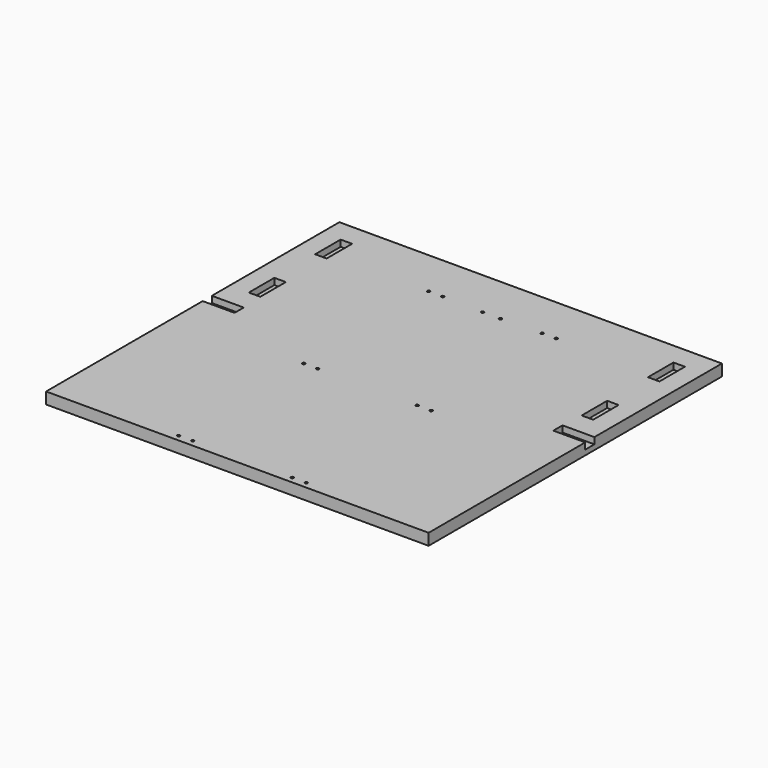
from build123d import *

# Parameters (mm, degrees)
F0_W     = 600
F0_H     = 575
F1_DEPTH = 18
F2_W     = 18
F2_H     = 50
F2_W_2   = 50
F2_H_2   = 18
F3_DEPTH = 10
F5_D     = 4.3
F6_D     = 4.3


with BuildPart() as f1:
    # F0 (on Top) → F1 (new body)
    with BuildSketch(Plane.XY):
        with Locations((300, -287.5)):
            Rectangle(F0_W, F0_H)
    extrude(amount=F1_DEPTH)

    # F2 (on face) → F3 (cut)
    with BuildSketch(Plane.XY.offset(18)):
        with Locations((39, -60)):
            Rectangle(F2_W, F2_H)
        with Locations((561, -60)):
            Rectangle(F2_W, F2_H)
        with Locations((561, -190)):
            Rectangle(F2_W, F2_H)
        with Locations((575, -259)):
            Rectangle(F2_W_2, F2_H_2)
        with Locations((25, -259)):
            Rectangle(F2_W_2, F2_H_2)
        with Locations((39, -190)):
            Rectangle(F2_W, F2_H)
    extrude(amount=-F3_DEPTH, mode=Mode.SUBTRACT)

    # F5 (through all)
    with Locations(Plane.XY.offset(18)):
        with Locations((200, -75), (222, -75), (200, -320), (222, -320), (378, -75), (400, -75), (400, -320), (378, -320), (378, -565), (400, -565), (200, -565), (222, -565)):
            Hole(F5_D / 2)

    # F6 (through all)
    with Locations(Plane.XY.offset(18)):
        with Locations((286, -76.75982), (314, -76.75982)):
            Hole(F6_D / 2)


solid = f1.part
